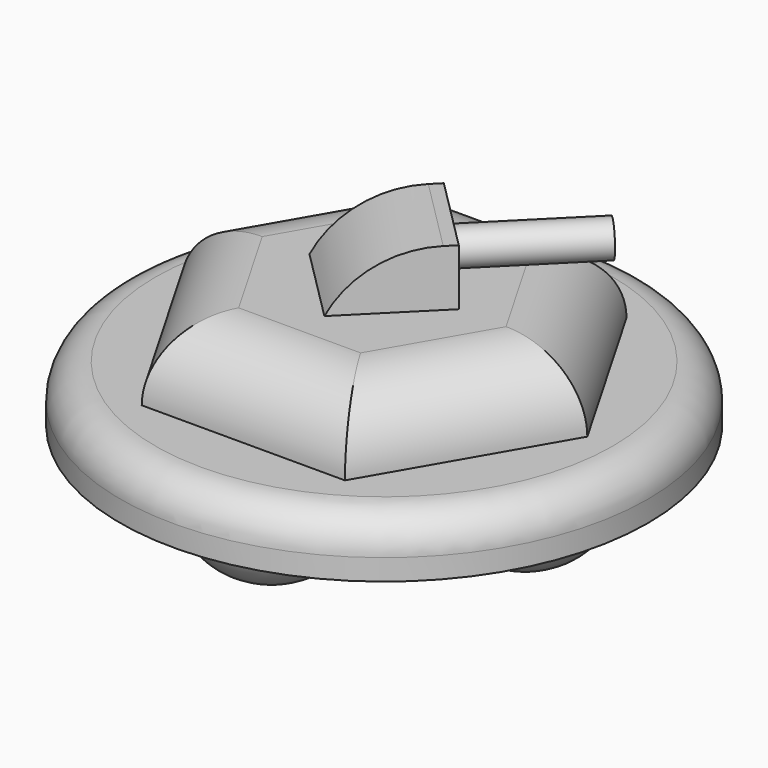
from build123d import *

# Parameters (mm, degrees)
F0_R         = 37.5
F1_DEPTH     = 8
F2_R         = 5
F3_R         = 11
F4_DEPTH     = 10
F5_R         = 9.99999
F7_DEPTH     = 10
F8_R         = 9.99999
F10_DEPTH    = 18
F11_T1_DEPTH = 81.3324958071
F12_R        = 2.5
F13_DEPTH    = 18


# Not quite as in the source:
# - a fillet or chamfer that OpenCascade refuses, or shapes differently, is made with other operations: its cross-section is extruded or revolved along the edge and cut away or added
# - a fillet or chamfer is up to 0.001 mm smaller than in the source, because OpenCascade refuses the exact size


with BuildPart() as f1:
    # F0 (on Top) → F1 (new body)
    with BuildSketch(Plane.XY):
        Circle(F0_R)
    extrude(amount=F1_DEPTH)

    # F2
    f2_edges = [f1.edges().sort_by_distance(p)[0] for p in [
        (-37.5, 0, 8),
    ]]
    fillet(f2_edges, radius=F2_R)

    # F3 (on face) → F4 (join)
    with BuildSketch(Plane(origin=(0, 0, 0), x_dir=(1, 0, 0), z_dir=(0, 0, -1))):
        with Locations((20, 0)):
            Circle(F3_R)
        with Locations((-20, 0)):
            Circle(F3_R)
        with Locations((0, 20)):
            Circle(F3_R)
        with Locations((0, -20)):
            Circle(F3_R)
    extrude(amount=F4_DEPTH)

    # F5 (radius 10 in the source; OpenCascade refuses exactly that, so slightly less here)
    f5_edges = [f1.edges().sort_by_distance(p)[0] for p in [
        (-11, 20, -10),
        (-31, 0, -10),
        (-11, -20, -10),
        (9, 0, -10),
    ]]
    fillet(f5_edges, radius=F5_R)

    # F6 (on face) → F7 (join)
    with BuildSketch(Plane.XY.offset(8)):
        Polygon((14.4337567297, -25), (28.8675134595, 0), (14.4337567297, 25), (-14.4337567297, 25), (-28.8675134595, 0), (-14.4337567297, -25), align=None)
    extrude(amount=F7_DEPTH)

    # F8 (radius 10 in the source; OpenCascade refuses exactly that, so slightly less here)
    f8_edges = [f1.edges().sort_by_distance(p)[0] for p in [
        (0, -25, 18),
        (21.650635, -12.5, 18),
        (21.650635, 12.5, 18),
        (0, 25, 18),
        (-21.650635, 12.5, 18),
        (-21.650635, -12.5, 18),
    ]]
    fillet(f8_edges, radius=F8_R)

    # F9 (on face) → F10 (join)
    with BuildSketch(Plane.XY.offset(8)):
        Polygon((10.6066017178, 0), (0, 10.6066017178), (-10.6066017178, 0), (0, -10.6066017178), align=None)
    extrude(amount=F10_DEPTH)

    # F11: fillet of radius 15 on 1 edges, made by hand

    # F11_s2 → F11_t1 (cut)
    with BuildSketch(Plane(origin=(-28.755379658, 28.755379658, 0), x_dir=(0, 0, 1), z_dir=(0.7071067812, -0.7071067812, 0))):
        with BuildLine():
            ThreePointArc((18, 7.5), (23.8452325787, 1.979467531), (26, -5.7664991614))
            Line((26, -5.7664991614), (26, 7.5))
            Line((26, 7.5), (18, 7.5))
        make_face()
    extrude(amount=F11_T1_DEPTH, mode=Mode.SUBTRACT)

    # F12 (on face) → F13 (join)
    with BuildSketch(Plane(origin=(5.3033008589, 5.3033008589, 0), x_dir=(-0.7071067812, 0.7071067812, 0), z_dir=(0.7071067812, 0.7071067812, 0))):
        with Locations((0, 22)):
            Circle(F12_R)
    extrude(amount=F13_DEPTH)


solid = f1.part
